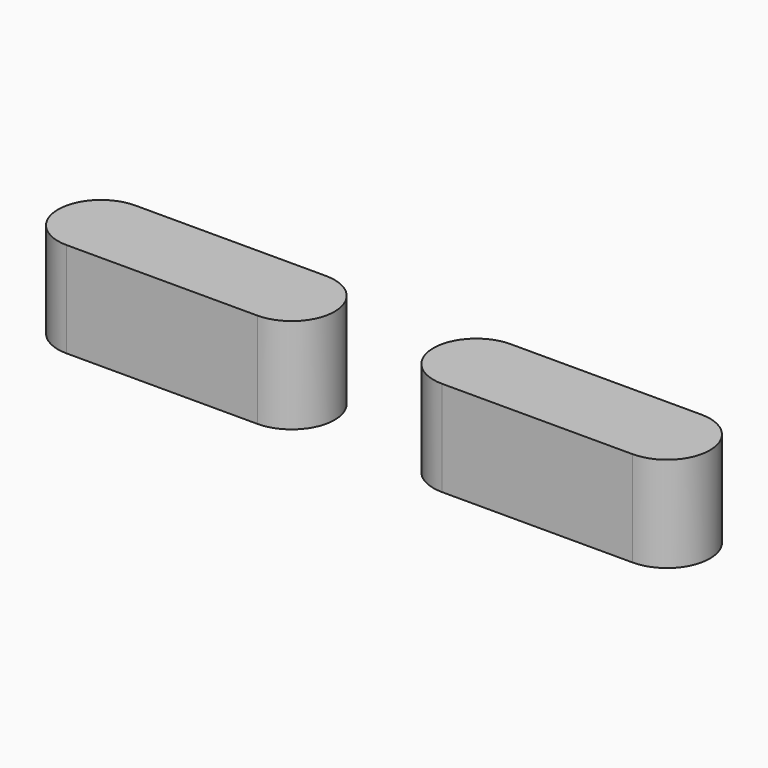
from build123d import *

# Parameters (mm, degrees)
F1_DEPTH = 20
F2_R     = 8.125
F3_DEPTH = 2
F4_DEPTH = 19


# Not quite as in the source:
# - a feature names something its author has since deleted; it is built from what else it names


with BuildPart() as f1:
    # F0 (on Top) → F1 (new body)
    with BuildSketch(Plane.XY):
        with BuildLine():
            Line((20, 9), (-20, 9))
            ThreePointArc((-20, 9), (-29, 0), (-20, -9))
            Line((-20, -9), (20, -9))
            ThreePointArc((20, -9), (29, 0), (20, 9))
        make_face()
    extrude(amount=F1_DEPTH)

    # F2 (on face) → F3 (cut)
    with BuildSketch(Plane(origin=(0, 0, 0), x_dir=(1, 0, 0), z_dir=(0, 0, -1))):
        with Locations((-20, 0)):
            Circle(F2_R)
        with Locations((20, 0)):
            Circle(F2_R)
    extrude(amount=-F3_DEPTH, mode=Mode.SUBTRACT)

    # F2 (on face) → F4 (cut)
    with BuildSketch(Plane(origin=(0, 0, 0), x_dir=(1, 0, 0), z_dir=(0, 0, -1))):
        with BuildLine():
            Line((2.5, 8.5), (-2.5, 8.5))
            ThreePointArc((-2.5, 8.5), (-11, 0), (-2.5, -8.5))
            Line((-2.5, -8.5), (2.5, -8.5))
            ThreePointArc((2.5, -8.5), (11, 0), (2.5, 8.5))
        make_face()
    extrude(amount=-F4_DEPTH, mode=Mode.SUBTRACT)


with BuildPart() as f5_1:
    # F5: copy of F1
    add(f1.part.moved(Location((78.7, 0, 0))))


solid = Compound([f1.part, f5_1.part])
